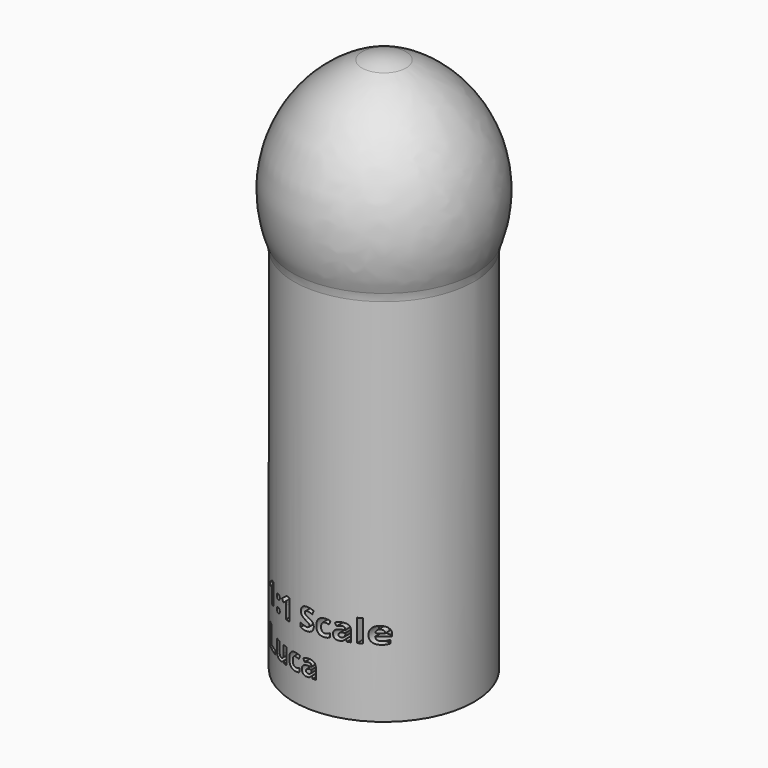
from build123d import *

# Parameters (mm, degrees)
F3_TEXT_SIZE = 6.5521023766
F4_DEPTH     = 25
F5_R         = 5


# Not quite as in the source:
# - Text() gives the source's letters only with a copy of the font that has no kerning and outlines rounded to 1/6400 em; it was checked with that copy


with BuildPart() as f1:
    # F0 (on Front) → F1 (revolve)
    with BuildSketch(Plane.XZ):
        with BuildLine():
            Line((0, 120), (0, 0))
            Line((0, 0), (20, 0))
            Line((20, 0), (20, 83.1489861012))
            ThreePointArc((20, 83.1489861012), (20.0053380987, 104.287405454), (4.8943040395, 119.0687941201))
            ThreePointArc((4.8943040395, 119.0687941201), (2.4910518071, 119.7651289648), (0, 120))
        make_face()
    revolve(axis=Axis((0, 0, 60), (0, 0, -1)))

    # F3 (on offset) → F4 (cut)
    with BuildSketch(Plane.XZ.offset(14.3)):
        with Locations((-14.0029789711, 15.1308167566)):
            Text('1:1 Scale', F3_TEXT_SIZE, font='Open Sans', font_style=FontStyle.BOLD, text_align=(TextAlign.LEFT, TextAlign.BOTTOM))
        with Locations((-14.0029789711, 6.2199575244)):
            Text('Luca', F3_TEXT_SIZE, font='Open Sans', font_style=FontStyle.BOLD, text_align=(TextAlign.LEFT, TextAlign.BOTTOM))
    extrude(amount=F4_DEPTH, mode=Mode.SUBTRACT)

    # F5
    f5_edges = [f1.edges().sort_by_distance(p)[0] for p in [
        (-20, 0, 83.148986),
    ]]
    fillet(f5_edges, radius=F5_R)


solid = f1.part
